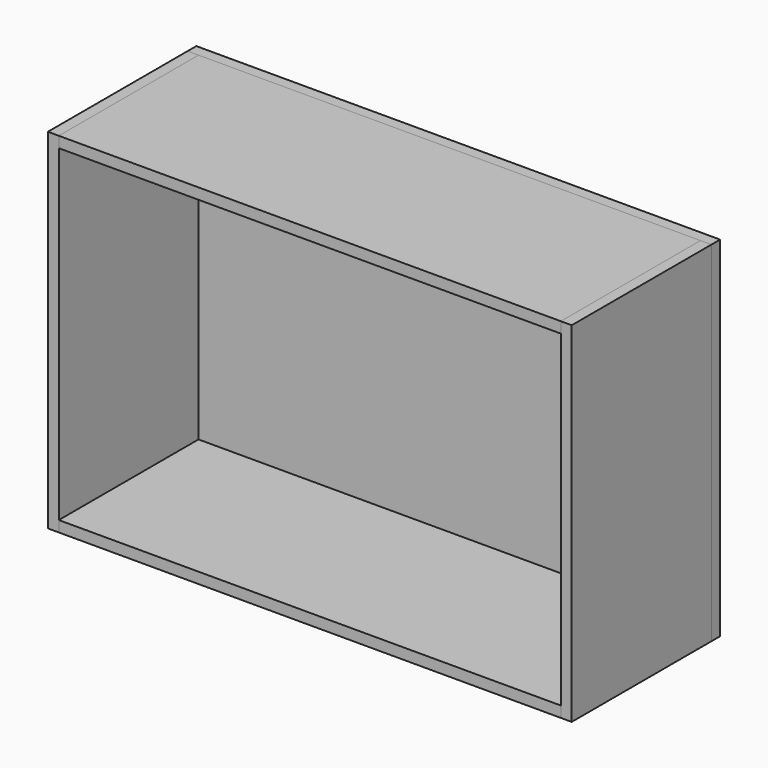
from build123d import *

# Parameters (mm, degrees)
F0_W     = 914.4
F0_H     = 609.6
F1_DEPTH = 19.05
F3_DEPTH = 304.8
F2_W     = 876.3
F2_H     = 19.05
F4_DEPTH = 304.8
F5_DEPTH = 304.8
F6_DEPTH = 304.8


with BuildPart() as f1:
    # F0 (on Front) → F1 (new body)
    with BuildSketch(Plane.XZ):
        Rectangle(F0_W, F0_H)
    extrude(amount=F1_DEPTH)


with BuildPart() as f3:
    # F2 (on face) → F3 (new body)
    with BuildSketch(Plane.XZ.offset(19.05)):
        Polygon((-457.2, 304.8), (-457.2, -304.8), (-438.15, -304.8), (-438.15, -285.75), (-438.15, 285.75), (-438.15, 304.8), align=None)
    extrude(amount=F3_DEPTH)


with BuildPart() as f4:
    # F2 (on face) → F4 (new body, through all)
    with BuildSketch(Plane.XZ.offset(19.05)):
        with Locations((0, -295.275)):
            Rectangle(F2_W, F2_H)
    extrude(amount=F4_DEPTH)


with BuildPart() as f5:
    # F2 (on face) → F5 (new body, through all)
    with BuildSketch(Plane.XZ.offset(19.05)):
        with Locations((0, 295.275)):
            Rectangle(F2_W, F2_H)
    extrude(amount=F5_DEPTH)


with BuildPart() as f6:
    # F2 (on face) → F6 (new body, through all)
    with BuildSketch(Plane.XZ.offset(19.05)):
        Polygon((438.15, -285.75), (438.15, -304.8), (457.2, -304.8), (457.2, 304.8), (438.15, 304.8), (438.15, 285.75), align=None)
    extrude(amount=F6_DEPTH)


solid = Compound([f1.part, f3.part, f4.part, f5.part, f6.part])
